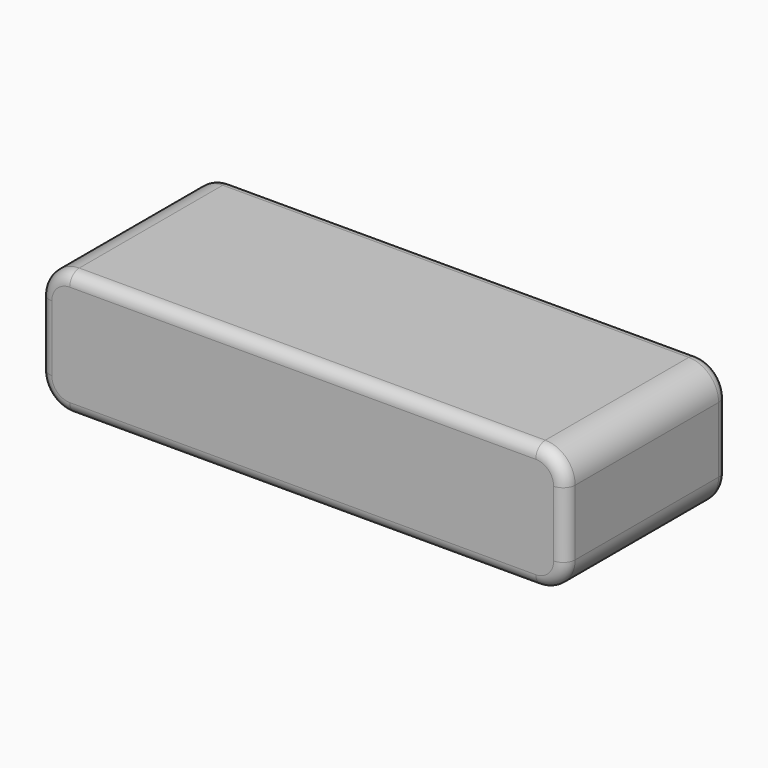
from build123d import *

# Parameters (mm, degrees)
F0_W         = 88
F0_H         = 34
F1_DEPTH     = 21
F2_R         = 2
F3_T1_DEPTH  = 34
F3_T4_ANGLE  = 90
F3_T6_ANGLE  = 90
F3_T8_ANGLE  = 90
F3_T10_ANGLE = 90
F3_T12_ANGLE = 90
F3_T14_ANGLE = 90
F3_T16_ANGLE = 90
F3_T18_ANGLE = 90


# Not quite as in the source:
# - a fillet or chamfer that OpenCascade refuses, or shapes differently, is made with other operations: its cross-section is extruded or revolved along the edge and cut away or added


with BuildPart() as f1:
    # F0 (on Top) → F1 (new body)
    with BuildSketch(Plane.XY):
        Rectangle(F0_W, F0_H)
    extrude(amount=F1_DEPTH)

    # F2
    f2_edges = [f1.edges().sort_by_distance(p)[0] for p in [
        (0, -17, 21),
        (0, -17, 0),
        (0, 17, 21),
        (0, 17, 0),
        (-44, 17, 10.5),
        (-44, -17, 10.5),
        (44, 17, 10.5),
        (44, -17, 10.5),
    ]]
    fillet(f2_edges, radius=F2_R)

    # F3: fillet of radius 5 on 4 edges, made by hand

    # F3_s2 → F3_t1 (cut)
    with BuildSketch(Plane.XZ.offset(-17)):
        with BuildLine():
            ThreePointArc((44, 5), (42.5355339059, 1.4644660941), (39, 0))
            Line((39, 0), (44, 0))
            Line((44, 0), (44, 5))
        make_face()
        with BuildLine():
            ThreePointArc((39, 21), (42.5355339059, 19.5355339059), (44, 16))
            Line((44, 16), (44, 21))
            Line((44, 21), (39, 21))
        make_face()
        with BuildLine():
            ThreePointArc((-44, 5), (-42.5355339059, 1.4644660941), (-39, 0))
            Line((-39, 0), (-44, 0))
            Line((-44, 0), (-44, 5))
        make_face()
        with BuildLine():
            ThreePointArc((-39, 21), (-42.5355339059, 19.5355339059), (-44, 16))
            Line((-44, 16), (-44, 21))
            Line((-44, 21), (-39, 21))
        make_face()
    extrude(amount=F3_T1_DEPTH, mode=Mode.SUBTRACT)

    # F3_s3 → F3_t4 (revolve, cut)
    with BuildSketch(Plane.XY.offset(16)):
        with BuildLine():
            ThreePointArc((-42, 17), (-43.4142135624, 16.4142135624), (-44, 15))
            Line((-44, 15), (-44, 17))
            Line((-44, 17), (-42, 17))
        make_face()
    revolve(axis=Axis((-39, 17, 16), (0, 1, 0)), revolution_arc=F3_T4_ANGLE, mode=Mode.SUBTRACT)

    # F3_s5 → F3_t6 (revolve, cut)
    with BuildSketch(Plane.YZ.offset(-39)):
        with BuildLine():
            ThreePointArc((-17, 19), (-16.4142135624, 20.4142135624), (-15, 21))
            Line((-15, 21), (-17, 21))
            Line((-17, 21), (-17, 19))
        make_face()
    revolve(axis=Axis((-39, -17, 16), (0, -1, 0)), revolution_arc=F3_T6_ANGLE, mode=Mode.SUBTRACT)

    # F3_s7 → F3_t8 (revolve, cut)
    with BuildSketch(Plane.YZ.offset(-39)):
        with BuildLine():
            ThreePointArc((17, 2), (16.4142135624, 0.5857864376), (15, 0))
            Line((15, 0), (17, 0))
            Line((17, 0), (17, 2))
        make_face()
    revolve(axis=Axis((-39, 17, 5), (0, 1, 0)), revolution_arc=F3_T8_ANGLE, mode=Mode.SUBTRACT)

    # F3_s9 → F3_t10 (revolve, cut)
    with BuildSketch(Plane.XY.offset(5)):
        with BuildLine():
            ThreePointArc((-42, -17), (-43.4142135624, -16.4142135624), (-44, -15))
            Line((-44, -15), (-44, -17))
            Line((-44, -17), (-42, -17))
        make_face()
    revolve(axis=Axis((-39, -17, 5), (0, -1, 0)), revolution_arc=F3_T10_ANGLE, mode=Mode.SUBTRACT)

    # F3_s11 → F3_t12 (revolve, cut)
    with BuildSketch(Plane.XY.offset(16)):
        with BuildLine():
            ThreePointArc((42, -17), (43.4142135624, -16.4142135624), (44, -15))
            Line((44, -15), (44, -17))
            Line((44, -17), (42, -17))
        make_face()
    revolve(axis=Axis((39, -17, 16), (0, -1, 0)), revolution_arc=F3_T12_ANGLE, mode=Mode.SUBTRACT)

    # F3_s13 → F3_t14 (revolve, cut)
    with BuildSketch(Plane.YZ.offset(39)):
        with BuildLine():
            ThreePointArc((17, 19), (16.4142135624, 20.4142135624), (15, 21))
            Line((15, 21), (17, 21))
            Line((17, 21), (17, 19))
        make_face()
    revolve(axis=Axis((39, 17, 16), (0, 1, 0)), revolution_arc=F3_T14_ANGLE, mode=Mode.SUBTRACT)

    # F3_s15 → F3_t16 (revolve, cut)
    with BuildSketch(Plane.YZ.offset(39)):
        with BuildLine():
            ThreePointArc((-17, 2), (-16.4142135624, 0.5857864376), (-15, 0))
            Line((-15, 0), (-17, 0))
            Line((-17, 0), (-17, 2))
        make_face()
    revolve(axis=Axis((39, -17, 5), (0, -1, 0)), revolution_arc=F3_T16_ANGLE, mode=Mode.SUBTRACT)

    # F3_s17 → F3_t18 (revolve, cut)
    with BuildSketch(Plane.XY.offset(5)):
        with BuildLine():
            ThreePointArc((42, 17), (43.4142135624, 16.4142135624), (44, 15))
            Line((44, 15), (44, 17))
            Line((44, 17), (42, 17))
        make_face()
    revolve(axis=Axis((39, 17, 5), (0, 1, 0)), revolution_arc=F3_T18_ANGLE, mode=Mode.SUBTRACT)


solid = f1.part
